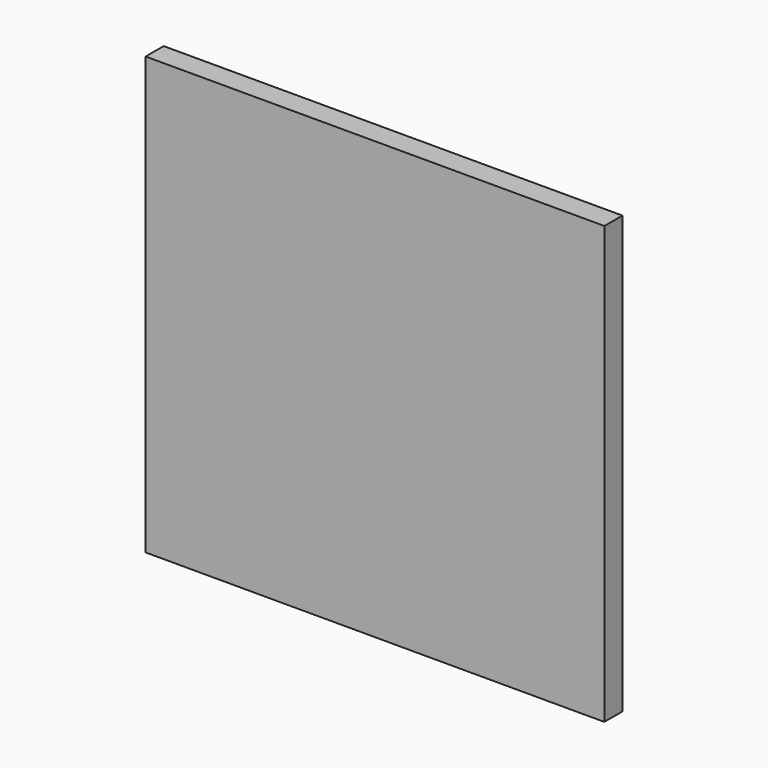
from build123d import *

# Parameters (mm, degrees)
F0_W     = 100
F0_H     = 86.7424257066
F2_DEPTH = 50
F1_W     = 1016
F1_H     = 966.9476541734
F3_T     = -2.5


# Not quite as in the source:
# - a feature names something its author has since deleted; it is built from what else it names


with BuildPart() as f2:
    # F0 (on Front) → F2 (new body)
    with BuildSketch(Plane.XZ):
        with Locations((7.0976624265, -4.7932257876)):
            Rectangle(F0_W, F0_H)
    extrude(amount=F2_DEPTH)

    # F3
    f3_openings = [f2.faces().sort_by_distance(p)[0] for p in [
        (7.097662, -50, -4.793226),
    ]]
    offset(amount=F3_T, openings=f3_openings)


with BuildPart() as f2b:
    # F1 (on face) → F2, piece 2 (new body)
    with BuildSketch(Plane.XZ):
        with Locations((0, -24.5261729133)):
            Rectangle(F1_W, F1_H)
    extrude(amount=F2_DEPTH)


solid = Compound([f2.part, f2b.part])
